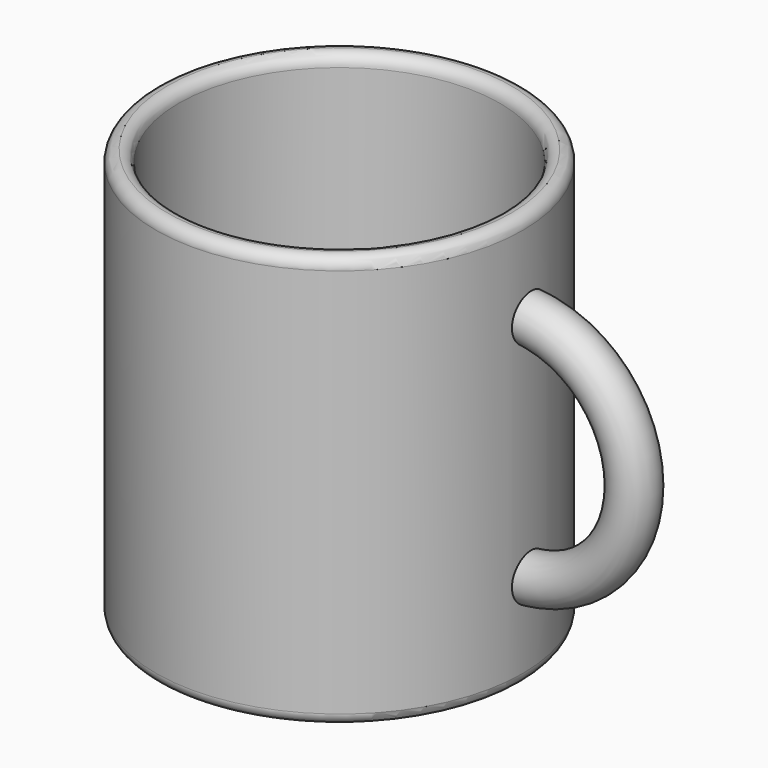
from build123d import *

# Parameters (mm, degrees)
F0_R         = 40
F1_DEPTH     = 90
F2_T         = -5
F4_R         = 5
F5_ANGLE     = 180
F6_R         = 2.49999
F7_TEXT_SIZE = 20.2835246455
F8_DEPTH     = 2.5


# Not quite as in the source:
# - a fillet or chamfer is up to 0.001 mm smaller than in the source, because OpenCascade refuses the exact size
# - Text() gives the source's letters only with a copy of the font that has no kerning and outlines rounded to 1/6400 em; it was checked with that copy


with BuildPart() as f1:
    # F0 (on Top) → F1 (new body)
    with BuildSketch(Plane.XY):
        with Locations((0, -2.1344509441)):
            Circle(F0_R)
    extrude(amount=F1_DEPTH)

    # F2
    f2_openings = [f1.faces().sort_by_distance(p)[0] for p in [
        (0, -2.134451, 90),
    ]]
    offset(amount=F2_T, openings=f2_openings)

    # F4 (on offset) → F5 (revolve)
    with BuildSketch(Plane.YZ.offset(37.5)):
        with Locations((0, 70)):
            Circle(F4_R)
    revolve(axis=Axis((37.5, 12.2337732464, 45), (0, 1, 0)), revolution_arc=F5_ANGLE)

    # F6 (radius 2.5 in the source; OpenCascade refuses exactly that, so slightly less here)
    f6_edges = [f1.edges().sort_by_distance(p)[0] for p in [
        (-40, -2.134451, 90),
        (-35, -2.134451, 90),
        (-40, -2.134451, 0),
    ]]
    fillet(f6_edges, radius=F6_R)

    # F7 (on face) → F8 (cut)
    with BuildSketch(Plane(origin=(0, 0, 0), x_dir=(1, 0, 0), z_dir=(0, 0, -1))):
        with Locations((-36.6496182582, -5.8062972277)):
            Text('TOMBE', F7_TEXT_SIZE, font='Open Sans', font_style=FontStyle.BOLD, text_align=(TextAlign.LEFT, TextAlign.BOTTOM))
    extrude(amount=-F8_DEPTH, mode=Mode.SUBTRACT)


solid = f1.part
